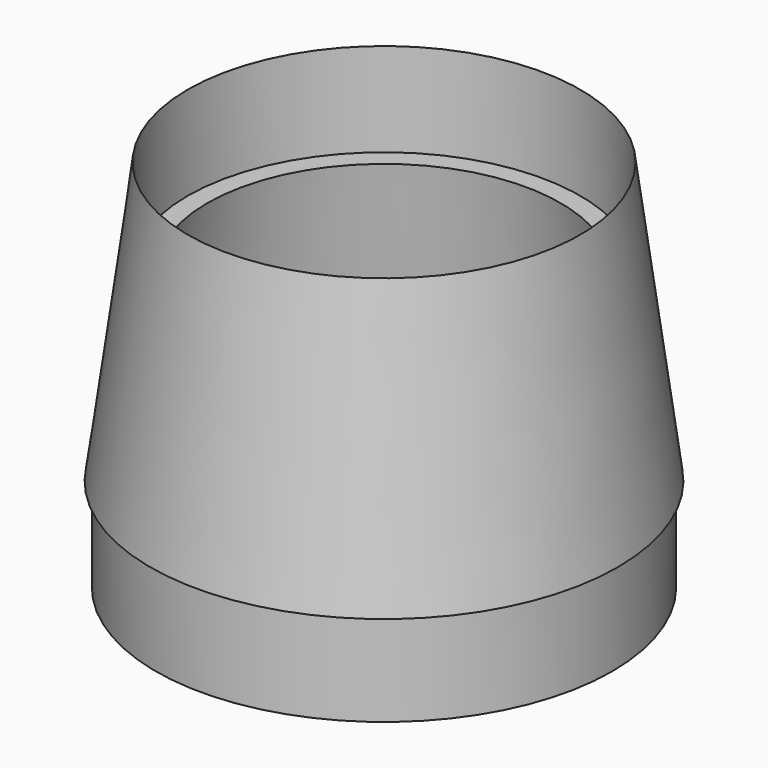
from build123d import *


# Not quite as in the source:
# - a feature names something its author has since deleted; it is built from what else it names


with BuildPart() as f1:
    # F0 (on Front) → F1 (revolve)
    with BuildSketch(Plane.XZ):
        Polygon((-24.4, 10), (-24.4, 0), (-22.9, 0), (-18.9, 30), (-21, 30), (-21, 40), (-25, 10), align=None)
    revolve(axis=Axis((0, 0, 20), (0, 0, 1)))


solid = f1.part
